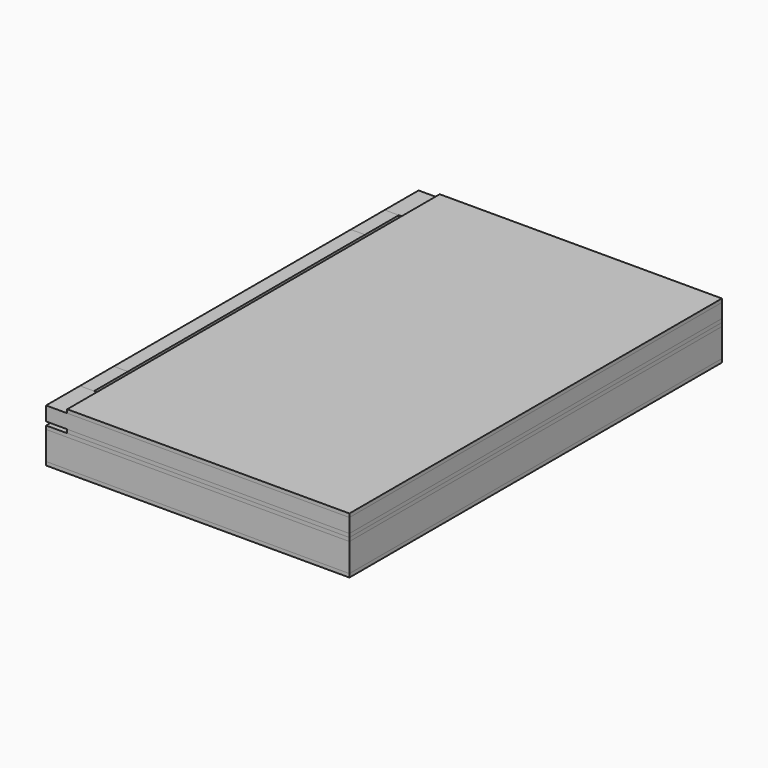
from build123d import *

# Parameters (mm, degrees)
F0_W      = 215
F0_H      = 330
F1_DEPTH  = 2.5
F2_W      = 215
F2_H      = 330
F2_W_2    = 195
F2_H_2    = 310
F3_DEPTH  = 20
F5_DEPTH  = 30
F8_W      = 215
F8_H      = 330
F9_DEPTH  = 2.5
F11_W     = 200
F11_H     = 330
F11_W_2   = 170
F11_H_2   = 300
F12_DEPTH = 2.5
F13_W     = 180
F13_H     = 310
F14_DEPTH = 10
F15_W     = 200
F15_H     = 330
F16_DEPTH = 2.5
F18_DEPTH = 210
F19_R     = 2
F20_DEPTH = 20
F21_R     = 2.5
F22_DEPTH = 5
F23_R     = 2
F24_DEPTH = 7.5
F25_R     = 2.5
F26_DEPTH = 10
F27_R     = 2
F28_DEPTH = 10
F29_DEPTH = 15
F30_R     = 2
F31_DEPTH = 30
F33_ANGLE = 17
F36_R     = 2.5
F37_DEPTH = 20
F38_R     = 2.5
F39_DEPTH = 15


with BuildPart() as f1:
    # F0 (on Top) → F1 (new body)
    with BuildSketch(Plane.XY):
        with Locations((107.5, 165)):
            Rectangle(F0_W, F0_H)
    extrude(amount=F1_DEPTH)


with BuildPart() as f3:
    # F2 (on face) → F3 (new body)
    with BuildSketch(Plane.XY.offset(2.5)):
        with Locations((107.5, 165)):
            Rectangle(F2_W, F2_H)
        with Locations((107.5, 165)):
            Rectangle(F2_W_2, F2_H_2, mode=Mode.SUBTRACT)
    extrude(amount=F3_DEPTH)


with BuildPart() as f5:
    # F4 (on Front) → F5 (new body)
    with BuildSketch(Plane.XZ):
        Polygon((0, 2.5), (0, 0), (0, -2.5), (10, -2.5), (10, 37.5), (0, 37.5), (0, 22.5), (5, 22.5), (5, 2.5), align=None)
    extrude(amount=-F5_DEPTH)


with BuildPart() as f5_1:
    # F6: moved
    add(f5.part.moved(Location((0, 30, 0))))


with BuildPart() as f7_1:
    # F7: copy of F5
    add(f5_1.part.moved(Location((0, 240, 0))))


with BuildPart() as f9:
    # F8 (on face) → F9 (new body)
    with BuildSketch(Plane.XY.offset(22.5)):
        with Locations((107.5, 165)):
            Rectangle(F8_W, F8_H)
    extrude(amount=F9_DEPTH)

    # F10: cut F7_1, F5
    add(f7_1.part, mode=Mode.SUBTRACT)
    add(f5_1.part, mode=Mode.SUBTRACT)


with BuildPart() as f3_1:
    add(f3.part)

    # F10: cut F7_1, F5
    add(f7_1.part, mode=Mode.SUBTRACT)
    add(f5_1.part, mode=Mode.SUBTRACT)


with BuildPart() as f1_1:
    add(f1.part)

    # F10: cut F7_1, F5
    add(f7_1.part, mode=Mode.SUBTRACT)
    add(f5_1.part, mode=Mode.SUBTRACT)


with BuildPart() as f12:
    # F11 (on face) → F12 (new body)
    with BuildSketch(Plane.XY.offset(25)):
        with Locations((115, 165)):
            Rectangle(F11_W, F11_H)
        with Locations((115, 165)):
            Rectangle(F11_W_2, F11_H_2, mode=Mode.SUBTRACT)
    extrude(amount=F12_DEPTH)


with BuildPart() as f14:
    # F13 (on face) → F14 (new body)
    with BuildSketch(Plane.XY.offset(27.5)):
        Polygon((0, 0), (215, 0), (215, 330), (0, 330), (0, 300), (15, 300), (15, 30), (0, 30), align=None)
        with Locations((115, 165)):
            Rectangle(F13_W, F13_H, mode=Mode.SUBTRACT)
    extrude(amount=F14_DEPTH)

    # F19 (on face) → F20 (cut)
    with BuildSketch(Plane.YZ.offset(25)):
        with Locations((20, 32.5)):
            Circle(F19_R)
    extrude(amount=-F20_DEPTH, mode=Mode.SUBTRACT)

    # F21 (on face) → F22 (cut)
    with BuildSketch(Plane(origin=(0, 30, 0), x_dir=(-1, 0, 0), z_dir=(0, 1, 0))):
        with Locations((-5, 32.5)):
            Circle(F21_R)
    extrude(amount=-F22_DEPTH, mode=Mode.SUBTRACT)

    # F23 (on face) → F24 (cut)
    with BuildSketch(Plane(origin=(0, 25, 0), x_dir=(-1, 0, 0), z_dir=(0, 1, 0))):
        with Locations((-5, 32.5)):
            Circle(F23_R)
    extrude(amount=-F24_DEPTH, mode=Mode.SUBTRACT)

    # F38 (on face) → F39 (cut)
    with BuildSketch(Plane.XZ.offset(-300)):
        with Locations((5, 32.5)):
            Circle(F38_R)
    extrude(amount=-F39_DEPTH, mode=Mode.SUBTRACT)


with BuildPart() as f16:
    # F15 (on face) → F16 (new body)
    with BuildSketch(Plane.XY.offset(37.5)):
        with Locations((115, 165)):
            Rectangle(F15_W, F15_H)
    extrude(amount=F16_DEPTH)


with BuildPart() as f18:
    # F17 (on face) → F18 (new body, through all)
    with BuildSketch(Plane.XZ.offset(-270)):
        Polygon((10, 37.5), (0, 37.5), (0, 25), (1, 25), (1, 36.5), (9, 36.5), (9, 25), (10, 25), align=None)
    extrude(amount=F18_DEPTH)


with BuildPart() as f5_2:
    add(f5_1.part)

    # F25 (on face) → F26 (cut)
    with BuildSketch(Plane.XZ.offset(-30)):
        with Locations((5, 32.5)):
            Circle(F25_R)
    extrude(amount=-F26_DEPTH, mode=Mode.SUBTRACT)

    # F27 (on face) → F28 (cut)
    with BuildSketch(Plane.XZ.offset(-40)):
        with Locations((5, 32.5)):
            Circle(F27_R)
    extrude(amount=-F28_DEPTH, mode=Mode.SUBTRACT)


with BuildPart() as f29:
    # F29 (new): a face of the model
    f29_faces = [f5_2.part.faces().sort_by_distance(p)[0] for p in [
        (2.570711, 40, 32.5),
    ]]
    extrude(f29_faces, amount=F29_DEPTH)


with BuildPart() as f31:
    # F30 (on Top) → F31 (new body)
    with BuildSketch(Plane.XY):
        with Locations((0, -3.60091)):
            Circle(F30_R)
    extrude(amount=F31_DEPTH)


with BuildPart() as f31_1:
    # F32: moved
    add(f31.part.moved(Location((10, 50, 0))))


with BuildPart() as f31_2:
    # F33: moved
    add(f31_1.part.rotate(Axis((5, 15, 22.5), (0, -1, 0)), F33_ANGLE))


with BuildPart() as f31_3:
    # F34: moved
    add(f31_2.part.moved(Location((-2.6, 0, 1.4))))


with BuildPart() as f5_3:
    add(f5_2.part)

    # F35: cut F31
    add(f31_3.part, mode=Mode.SUBTRACT)


with BuildPart() as f7_1_1:
    add(f7_1.part)

    # F36 (on face) → F37 (cut)
    with BuildSketch(Plane(origin=(0, 300, 0), x_dir=(-1, 0, 0), z_dir=(0, 1, 0))):
        with Locations((-5, 32.5)):
            Circle(F36_R)
    extrude(amount=-F37_DEPTH, mode=Mode.SUBTRACT)


solid = Compound([f9.part, f3_1.part, f1_1.part, f12.part, f14.part, f16.part, f18.part, f29.part, f5_3.part, f7_1_1.part])
